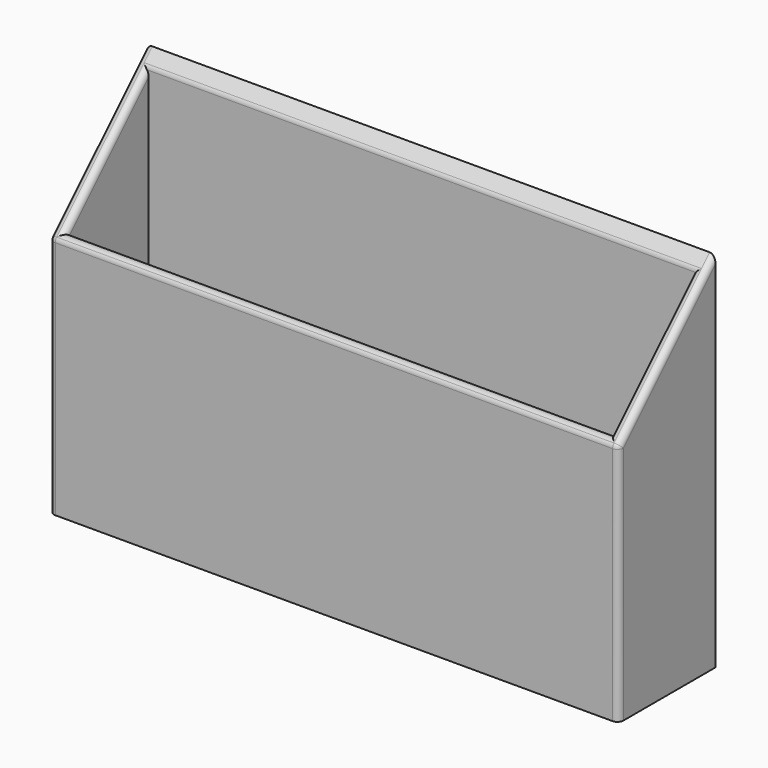
from build123d import *

# Parameters (mm, degrees)
F1_DEPTH = 59.65
F3_DEPTH = 57.15
F4_R     = 1.24999


# Not quite as in the source:
# - a fillet or chamfer is up to 0.001 mm smaller than in the source, because OpenCascade refuses the exact size


with BuildPart() as f1:
    # F0 (on Right) → F1 (new body, symmetric)
    with BuildSketch(Plane.YZ):
        Polygon((-25.4, 0), (0, 0), (0, 76.2), (-25.4, 50.8), align=None)
    extrude(amount=F1_DEPTH, both=True)

    # F2 (on Right) → F3 (cut, symmetric)
    with BuildSketch(Plane.YZ):
        Polygon((-2.5, 73.7), (-22.9, 53.3), (-22.9, 2.5), (-2.5, 2.5), align=None)
    extrude(amount=F3_DEPTH, both=True, mode=Mode.SUBTRACT)

    # F4 (radius 1.25 in the source; OpenCascade refuses exactly that, so slightly less here)
    f4_edges = [f1.edges().sort_by_distance(p)[0] for p in [
        (-59.65, -25.4, 25.4),
        (59.65, -25.4, 25.4),
        (59.65, -12.7, 63.5),
        (0, -25.4, 50.8),
        (-59.65, -12.7, 63.5),
        (57.15, -12.7, 63.5),
        (0, -22.9, 53.3),
        (0, -2.5, 73.7),
        (-57.15, -12.7, 63.5),
    ]]
    fillet(f4_edges, radius=F4_R)


solid = f1.part
